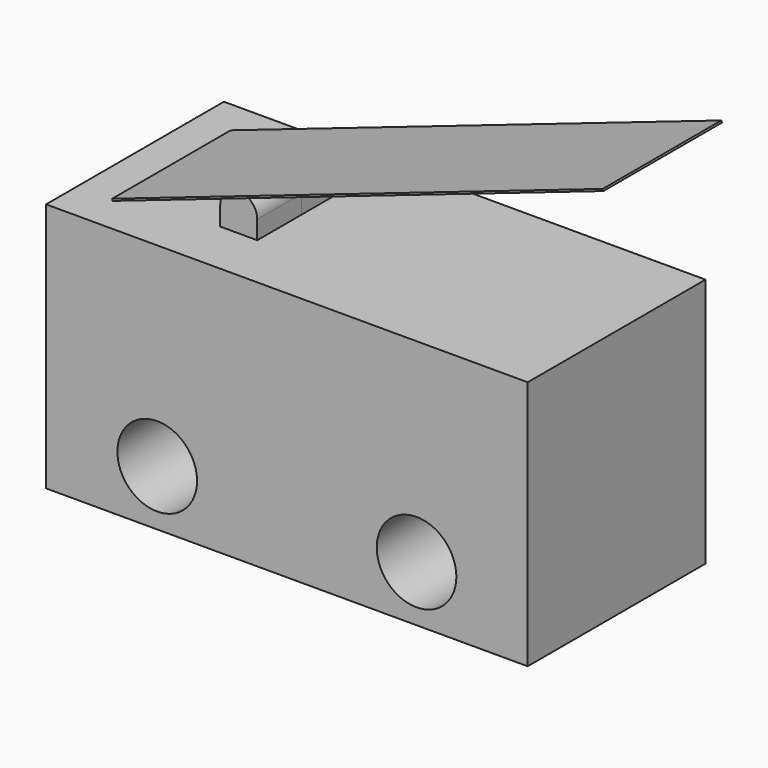
from build123d import *

# Parameters (mm, degrees)
F0_R     = 1.075
F1_DEPTH = 3
F2_DEPTH = 1.5
F3_DEPTH = 2


with BuildPart() as f1:
    # F0 (on Front) → F1 (new body, symmetric)
    with BuildSketch(Plane.XZ):
        Polygon((-12, 6.75), (-13, 6.75), (-13, 0), (0, 0), (0, 6.75), (-8.5, 6.75), (-9.5, 6.75), align=None)
        with Locations((-10, 1.5)):
            Circle(F0_R, mode=Mode.SUBTRACT)
        with Locations((-3, 1.5)):
            Circle(F0_R, mode=Mode.SUBTRACT)
    extrude(amount=F1_DEPTH, both=True)


with BuildPart() as f2:
    # F0 (on Front) → F2 (new body, symmetric)
    with BuildSketch(Plane.XZ):
        with BuildLine():
            Line((-9.5, 7.25), (-9.5, 6.75))
            Line((-9.5, 6.75), (-8.5, 6.75))
            Line((-8.5, 6.75), (-8.5, 7.25))
            ThreePointArc((-8.5, 7.25), (-8.7093808918, 7.6568667275), (-9.1621621359, 7.722972982))
            ThreePointArc((-9.1621621359, 7.722972982), (-9.4068667275, 7.5406191082), (-9.5, 7.25))
        make_face()
    extrude(amount=F2_DEPTH, both=True)


with BuildPart() as f3:
    # F0 (on Front) → F3 (new body, symmetric)
    with BuildSketch(Plane.XZ):
        Polygon((-12.0162162162, 6.7972972973), (-12, 6.75), (-9.1621621359, 7.722972982), (1.2432432432, 11.2905405405), (1.227027027, 11.3378378378), align=None)
    extrude(amount=F3_DEPTH, both=True)


solid = Compound([f1.part, f2.part, f3.part])
